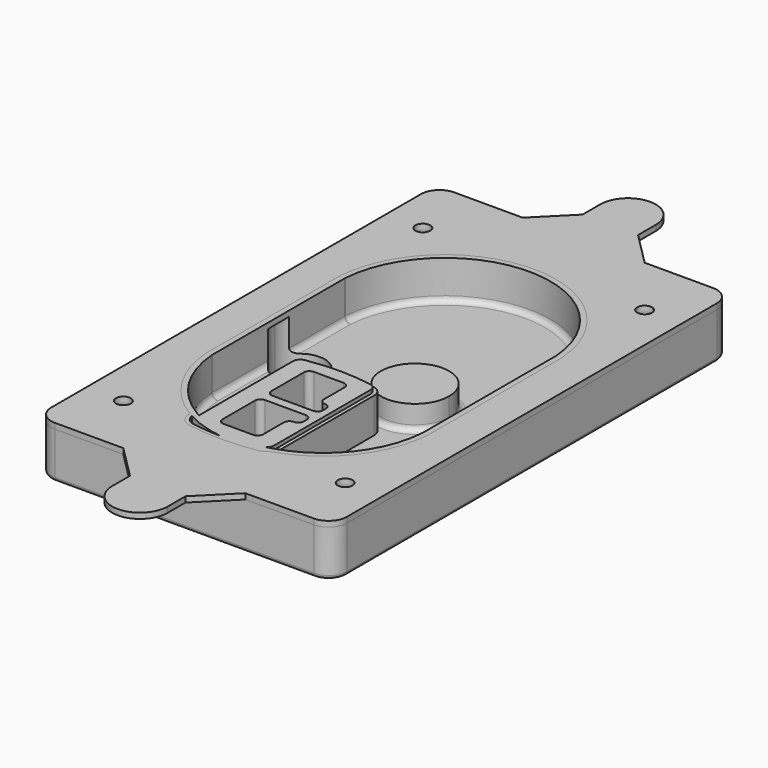
from build123d import *

# Parameters (mm, degrees)
F0_R      = 4
F1_DEPTH  = 25
F2_DEPTH  = 3
F3_DEPTH  = 18
F6_DEPTH  = 2
F8_DEPTH  = 20
F9_DEPTH  = 16
F10_DEPTH = 25
F7_R      = 6
F7_R_2    = 4
F11_DEPTH = 6
F13_DEPTH = 9
F14_R     = 3
F15_R     = 2
F16_R     = 4
F16_R_2   = 6
F17_DEPTH = 3


with BuildPart() as f1:
    # F0 (on Top) → F1 (new body)
    with BuildSketch(Plane.XY):
        with BuildLine():
            ThreePointArc((14.05, 38.3825811321), (16.9789321881, 31.3115133202), (24.05, 28.3825811321))
            Line((24.05, 28.3825811321), (164.05, 28.3825811321))
            ThreePointArc((164.05, 28.3825811321), (171.1210678119, 31.3115133202), (174.05, 38.3825811321))
            Line((174.05, 38.3825811321), (174.05, 288.3825811321))
            ThreePointArc((174.05, 288.3825811321), (171.1210678119, 295.4536489439), (164.05, 298.3825811321))
            Line((164.05, 298.3825811321), (24.05, 298.3825811321))
            ThreePointArc((24.05, 298.3825811321), (16.9789321881, 295.4536489439), (14.05, 288.3825811321))
            Line((14.05, 288.3825811321), (14.05, 38.3825811321))
        make_face()
        with Locations((34.05, 62.1325811321)):
            Circle(F0_R, mode=Mode.SUBTRACT)
        with Locations((154.05, 62.1325811321)):
            Circle(F0_R, mode=Mode.SUBTRACT)
        with Locations((34.05, 264.6325811321)):
            Circle(F0_R, mode=Mode.SUBTRACT)
        with BuildLine():
            ThreePointArc((30.05, 208.0453240566), (30.058730902, 208.5396812427), (30.0849127182, 209.033421831))
            ThreePointArc((30.0849127182, 209.033421831), (94.05, 268.6325811321), (158.0150872818, 209.033421831))
            ThreePointArc((158.0150872818, 209.033421831), (158.041269098, 208.5396812427), (158.05, 208.0453240566))
            Line((158.05, 208.0453240566), (158.05, 118.7198382075))
            ThreePointArc((158.05, 118.7198382075), (158.041269098, 118.2254810215), (158.0150872818, 117.7317404331))
            ThreePointArc((158.0150872818, 117.7317404331), (94.05, 58.1325811321), (30.0849127182, 117.7317404331))
            ThreePointArc((30.0849127182, 117.7317404331), (30.058730902, 118.2254810215), (30.05, 118.7198382075))
            Line((30.05, 118.7198382075), (30.05, 208.0453240566))
        make_face(mode=Mode.SUBTRACT)
        with Locations((154.05, 264.6325811321)):
            Circle(F0_R, mode=Mode.SUBTRACT)
        with BuildLine():
            ThreePointArc((158.0150872818, 209.033421831), (94.05, 268.6325811321), (30.0849127182, 209.033421831))
            ThreePointArc((30.0849127182, 209.033421831), (30.058730902, 208.5396812427), (30.05, 208.0453240566))
            Line((30.05, 208.0453240566), (30.05, 118.7198382075))
            ThreePointArc((30.05, 118.7198382075), (30.058730902, 118.2254810215), (30.0849127182, 117.7317404331))
            ThreePointArc((30.0849127182, 117.7317404331), (94.05, 58.1325811321), (158.0150872818, 117.7317404331))
            ThreePointArc((158.0150872818, 117.7317404331), (158.041269098, 118.2254810215), (158.05, 118.7198382075))
            Line((158.05, 118.7198382075), (158.05, 208.0453240566))
            ThreePointArc((158.05, 208.0453240566), (158.041269098, 208.5396812427), (158.0150872818, 209.033421831))
        make_face()
        with BuildLine():
            Line((34.05, 118.7198382075), (34.05, 208.0453240566))
            ThreePointArc((34.05, 208.0453240566), (34.0562363586, 208.3984363324), (34.0749376559, 208.7511081812))
            ThreePointArc((34.0749376559, 208.7511081812), (94.05, 264.6325811321), (154.0250623441, 208.7511081812))
            ThreePointArc((154.0250623441, 208.7511081812), (154.0437636414, 208.3984363324), (154.05, 208.0453240566))
            Line((154.05, 208.0453240566), (154.05, 118.7198382075))
            ThreePointArc((154.05, 118.7198382075), (154.0437636414, 118.3667259318), (154.0250623441, 118.0140540829))
            ThreePointArc((154.0250623441, 118.0140540829), (94.05, 62.1325811321), (34.0749376559, 118.0140540829))
            ThreePointArc((34.0749376559, 118.0140540829), (34.0562363586, 118.3667259318), (34.05, 118.7198382075))
        make_face(mode=Mode.SUBTRACT)
        with BuildLine():
            ThreePointArc((34.0749376559, 208.7511081812), (34.0562363586, 208.3984363324), (34.05, 208.0453240566))
            Line((34.05, 208.0453240566), (34.05, 118.7198382075))
            ThreePointArc((34.05, 118.7198382075), (34.0562363586, 118.3667259318), (34.0749376559, 118.0140540829))
            ThreePointArc((34.0749376559, 118.0140540829), (94.05, 62.1325811321), (154.0250623441, 118.0140540829))
            ThreePointArc((154.0250623441, 118.0140540829), (154.0437636414, 118.3667259318), (154.05, 118.7198382075))
            Line((154.05, 118.7198382075), (154.05, 208.0453240566))
            ThreePointArc((154.05, 208.0453240566), (154.0437636414, 208.3984363324), (154.0250623441, 208.7511081812))
            ThreePointArc((154.0250623441, 208.7511081812), (94.05, 264.6325811321), (34.0749376559, 208.7511081812))
        make_face()
        with BuildLine():
            ThreePointArc((151.0325436409, 208.5393729438), (151.045634549, 208.2925026496), (151.05, 208.0453240566))
            Line((151.05, 208.0453240566), (151.05, 118.7198382075))
            ThreePointArc((151.05, 118.7198382075), (151.045634549, 118.4726596145), (151.0325436409, 118.2257893203))
            ThreePointArc((151.0325436409, 118.2257893203), (94.05, 65.1325811321), (37.0674563591, 118.2257893203))
            ThreePointArc((37.0674563591, 118.2257893203), (37.054365451, 118.4726596145), (37.05, 118.7198382075))
            Line((37.05, 118.7198382075), (37.05, 208.0453240566))
            ThreePointArc((37.05, 208.0453240566), (37.054365451, 208.2925026496), (37.0674563591, 208.5393729438))
            ThreePointArc((37.0674563591, 208.5393729438), (94.05, 261.6325811321), (151.0325436409, 208.5393729438))
        make_face(mode=Mode.SUBTRACT)
        with BuildLine():
            Line((151.05, 118.7198382075), (151.05, 208.0453240566))
            ThreePointArc((151.05, 208.0453240566), (151.045634549, 208.2925026496), (151.0325436409, 208.5393729438))
            ThreePointArc((151.0325436409, 208.5393729438), (94.05, 261.6325811321), (37.0674563591, 208.5393729438))
            ThreePointArc((37.0674563591, 208.5393729438), (37.054365451, 208.2925026496), (37.05, 208.0453240566))
            Line((37.05, 208.0453240566), (37.05, 118.7198382075))
            ThreePointArc((37.05, 118.7198382075), (37.054365451, 118.4726596145), (37.0674563591, 118.2257893203))
            ThreePointArc((37.0674563591, 118.2257893203), (94.05, 65.1325811321), (151.0325436409, 118.2257893203))
            ThreePointArc((151.0325436409, 118.2257893203), (151.045634549, 118.4726596145), (151.05, 118.7198382075))
        make_face()
    extrude(amount=-F1_DEPTH)

    # F0 (on Top) → F2 (join)
    with BuildSketch(Plane.XY):
        with BuildLine():
            ThreePointArc((34.0749376559, 208.7511081812), (34.0562363586, 208.3984363324), (34.05, 208.0453240566))
            Line((34.05, 208.0453240566), (34.05, 118.7198382075))
            ThreePointArc((34.05, 118.7198382075), (34.0562363586, 118.3667259318), (34.0749376559, 118.0140540829))
            ThreePointArc((34.0749376559, 118.0140540829), (94.05, 62.1325811321), (154.0250623441, 118.0140540829))
            ThreePointArc((154.0250623441, 118.0140540829), (154.0437636414, 118.3667259318), (154.05, 118.7198382075))
            Line((154.05, 118.7198382075), (154.05, 208.0453240566))
            ThreePointArc((154.05, 208.0453240566), (154.0437636414, 208.3984363324), (154.0250623441, 208.7511081812))
            ThreePointArc((154.0250623441, 208.7511081812), (94.05, 264.6325811321), (34.0749376559, 208.7511081812))
        make_face()
        with BuildLine():
            ThreePointArc((151.0325436409, 208.5393729438), (151.045634549, 208.2925026496), (151.05, 208.0453240566))
            Line((151.05, 208.0453240566), (151.05, 118.7198382075))
            ThreePointArc((151.05, 118.7198382075), (151.045634549, 118.4726596145), (151.0325436409, 118.2257893203))
            ThreePointArc((151.0325436409, 118.2257893203), (94.05, 65.1325811321), (37.0674563591, 118.2257893203))
            ThreePointArc((37.0674563591, 118.2257893203), (37.054365451, 118.4726596145), (37.05, 118.7198382075))
            Line((37.05, 118.7198382075), (37.05, 208.0453240566))
            ThreePointArc((37.05, 208.0453240566), (37.054365451, 208.2925026496), (37.0674563591, 208.5393729438))
            ThreePointArc((37.0674563591, 208.5393729438), (94.05, 261.6325811321), (151.0325436409, 208.5393729438))
        make_face(mode=Mode.SUBTRACT)
    extrude(amount=F2_DEPTH)

    # F0 (on Top) → F3 (cut)
    with BuildSketch(Plane.XY):
        with BuildLine():
            Line((151.05, 118.7198382075), (151.05, 208.0453240566))
            ThreePointArc((151.05, 208.0453240566), (151.045634549, 208.2925026496), (151.0325436409, 208.5393729438))
            ThreePointArc((151.0325436409, 208.5393729438), (94.05, 261.6325811321), (37.0674563591, 208.5393729438))
            ThreePointArc((37.0674563591, 208.5393729438), (37.054365451, 208.2925026496), (37.05, 208.0453240566))
            Line((37.05, 208.0453240566), (37.05, 118.7198382075))
            ThreePointArc((37.05, 118.7198382075), (37.054365451, 118.4726596145), (37.0674563591, 118.2257893203))
            ThreePointArc((37.0674563591, 118.2257893203), (94.05, 65.1325811321), (151.0325436409, 118.2257893203))
            ThreePointArc((151.0325436409, 118.2257893203), (151.045634549, 118.4726596145), (151.05, 118.7198382075))
        make_face()
    extrude(amount=-F3_DEPTH, mode=Mode.SUBTRACT)

    # F4 (on face) → F5 (join, up to the next surface of F1)
    with BuildSketch(Plane.XY.offset(3)):
        with BuildLine():
            ThreePointArc((63.3, 70.0663530628), (65.1877495215, 64.9049197262), (69.9600985222, 62.1793597175))
            ThreePointArc((69.9600985222, 62.1793597175), (88.3, 60.6325811321), (106.6399014778, 62.1793597175))
            ThreePointArc((106.6399014778, 62.1793597175), (109.0997725506, 63.0263439319), (111.1577970177, 64.617847387))
            ThreePointArc((111.1577970177, 64.617847387), (98.7563887447, 62.3170645345), (86.1478631202, 62.6541260499))
            ThreePointArc((86.1478631202, 62.6541260499), (78.1937130529, 63.1086914432), (70.2950738916, 64.1511080538))
            ThreePointArc((70.2950738916, 64.1511080538), (66.9266219225, 65.9586086463), (65.3334610334, 69.4335712996))
            ThreePointArc((65.3334610334, 69.4335712996), (64.3111007877, 70.0023086838), (63.3, 70.5908304601))
            Line((63.3, 70.5908304601), (63.3, 70.0663530628))
        make_face()
        with BuildLine():
            ThreePointArc((107.5304157815, 66.7459245602), (109.1654742984, 67.168670617), (110.7873217221, 67.6395649966))
            ThreePointArc((110.7873217221, 67.6395649966), (111.1704314293, 68.826177739), (111.3, 70.0663530628))
            Line((111.3, 70.0663530628), (111.3, 135.1988092013))
            ThreePointArc((111.3, 135.1988092013), (109.8841878588, 139.0698842038), (106.3049261084, 141.1140542103))
            ThreePointArc((106.3049261084, 141.1140542103), (88.3, 142.6325811321), (70.2950738916, 141.1140542103))
            ThreePointArc((70.2950738916, 141.1140542103), (66.7158121412, 139.0698842038), (65.3, 135.1988092013))
            Line((65.3, 135.1988092013), (65.3, 72.8946079133))
            ThreePointArc((65.3, 72.8946079133), (66.2944325049, 72.3286907176), (67.3, 71.7828040152))
            Line((67.3, 71.7828040152), (67.3, 135.1988092013))
            ThreePointArc((67.3, 135.1988092013), (68.2438747608, 137.7795258696), (70.6300492611, 139.142305874))
            ThreePointArc((70.6300492611, 139.142305874), (88.3, 140.6325811321), (105.9699507389, 139.142305874))
            ThreePointArc((105.9699507389, 139.142305874), (108.3561252392, 137.7795258696), (109.3, 135.1988092013))
            Line((109.3, 135.1988092013), (109.3, 70.0663530628))
            ThreePointArc((109.3, 70.0663530628), (108.8299903064, 68.185085289), (107.5304157815, 66.7459245602))
        make_face()
        with BuildLine():
            ThreePointArc((67.3, 71.7828040152), (86.9533102792, 65.5751092381), (107.5304157815, 66.7459245602))
            ThreePointArc((107.5304157815, 66.7459245602), (108.8299903064, 68.185085289), (109.3, 70.0663530628))
            Line((109.3, 70.0663530628), (109.3, 135.1988092013))
            ThreePointArc((109.3, 135.1988092013), (108.3561252392, 137.7795258696), (105.9699507389, 139.142305874))
            ThreePointArc((105.9699507389, 139.142305874), (88.3, 140.6325811321), (70.6300492611, 139.142305874))
            ThreePointArc((70.6300492611, 139.142305874), (68.2438747608, 137.7795258696), (67.3, 135.1988092013))
            Line((67.3, 135.1988092013), (67.3, 71.7828040152))
        make_face()
        with BuildLine():
            Line((80.3, 100.1325811321), (102.3, 100.1325811321))
            ThreePointArc((102.3, 100.1325811321), (104.4213203436, 99.2539014756), (105.3, 97.1325811321))
            Line((105.3, 97.1325811321), (105.3, 95.1325811321))
            ThreePointArc((105.3, 95.1325811321), (104.4213203436, 93.0112607885), (102.3, 92.1325811321))
            ThreePointArc((102.3, 92.1325811321), (100.1786796564, 91.2539014756), (99.3, 89.1325811321))
            Line((99.3, 89.1325811321), (99.3, 75.1325811321))
            ThreePointArc((99.3, 75.1325811321), (98.4213203436, 73.0112607885), (96.3, 72.1325811321))
            Line((96.3, 72.1325811321), (80.3, 72.1325811321))
            ThreePointArc((80.3, 72.1325811321), (78.1786796564, 73.0112607885), (77.3, 75.1325811321))
            Line((77.3, 75.1325811321), (77.3, 97.1325811321))
            ThreePointArc((77.3, 97.1325811321), (78.1786796564, 99.2539014756), (80.3, 100.1325811321))
        make_face(mode=Mode.SUBTRACT)
        with BuildLine():
            ThreePointArc((80.3, 105.1325811321), (78.1786796564, 106.0112607885), (77.3, 108.1325811321))
            Line((77.3, 108.1325811321), (77.3, 130.1325811321))
            ThreePointArc((77.3, 130.1325811321), (78.1786796564, 132.2539014756), (80.3, 133.1325811321))
            Line((80.3, 133.1325811321), (96.3, 133.1325811321))
            ThreePointArc((96.3, 133.1325811321), (98.4213203436, 132.2539014756), (99.3, 130.1325811321))
            Line((99.3, 130.1325811321), (99.3, 116.1325811321))
            ThreePointArc((99.3, 116.1325811321), (100.1786796564, 114.0112607885), (102.3, 113.1325811321))
            ThreePointArc((102.3, 113.1325811321), (104.4213203436, 112.2539014756), (105.3, 110.1325811321))
            Line((105.3, 110.1325811321), (105.3, 108.1325811321))
            ThreePointArc((105.3, 108.1325811321), (104.4213203436, 106.0112607885), (102.3, 105.1325811321))
            Line((102.3, 105.1325811321), (80.3, 105.1325811321))
        make_face(mode=Mode.SUBTRACT)
    extrude(until=Until.NEXT, dir=(0, 0, -1))

    # F4 (on face) → F6 (cut)
    with BuildSketch(Plane.XY.offset(3)):
        with BuildLine():
            ThreePointArc((107.5304157815, 66.7459245602), (109.1654742984, 67.168670617), (110.7873217221, 67.6395649966))
            ThreePointArc((110.7873217221, 67.6395649966), (111.1704314293, 68.826177739), (111.3, 70.0663530628))
            Line((111.3, 70.0663530628), (111.3, 135.1988092013))
            ThreePointArc((111.3, 135.1988092013), (109.8841878588, 139.0698842038), (106.3049261084, 141.1140542103))
            ThreePointArc((106.3049261084, 141.1140542103), (88.3, 142.6325811321), (70.2950738916, 141.1140542103))
            ThreePointArc((70.2950738916, 141.1140542103), (66.7158121412, 139.0698842038), (65.3, 135.1988092013))
            Line((65.3, 135.1988092013), (65.3, 72.8946079133))
            ThreePointArc((65.3, 72.8946079133), (66.2944325049, 72.3286907176), (67.3, 71.7828040152))
            Line((67.3, 71.7828040152), (67.3, 135.1988092013))
            ThreePointArc((67.3, 135.1988092013), (68.2438747608, 137.7795258696), (70.6300492611, 139.142305874))
            ThreePointArc((70.6300492611, 139.142305874), (88.3, 140.6325811321), (105.9699507389, 139.142305874))
            ThreePointArc((105.9699507389, 139.142305874), (108.3561252392, 137.7795258696), (109.3, 135.1988092013))
            Line((109.3, 135.1988092013), (109.3, 70.0663530628))
            ThreePointArc((109.3, 70.0663530628), (108.8299903064, 68.185085289), (107.5304157815, 66.7459245602))
        make_face()
    extrude(amount=-F6_DEPTH, mode=Mode.SUBTRACT)

    # F7 (on face) → F8 (join)
    with BuildSketch(Plane(origin=(0, 0, -25), x_dir=(1, 0, 0), z_dir=(0, 0, -1))):
        with BuildLine():
            ThreePointArc((97.33842436, -163.3825811321), (110.8067035675, -149.9143019245), (124.274982775, -163.3825811321))
            Line((124.274982775, -163.3825811321), (129.274982775, -163.3825811321))
            ThreePointArc((129.274982775, -163.3825811321), (110.8067035675, -144.9143019245), (92.33842436, -163.3825811321))
            Line((92.33842436, -163.3825811321), (97.33842436, -163.3825811321))
        make_face()
        with BuildLine():
            Line((97.33842436, -163.3825811321), (124.274982775, -163.3825811321))
            ThreePointArc((124.274982775, -163.3825811321), (110.8067035675, -149.9143019245), (97.33842436, -163.3825811321))
        make_face()
        with BuildLine():
            ThreePointArc((97.33842436, -163.3825811321), (110.8067035675, -176.8508603396), (124.274982775, -163.3825811321))
            Line((124.274982775, -163.3825811321), (97.33842436, -163.3825811321))
        make_face()
        with BuildLine():
            Line((129.274982775, -163.3825811321), (124.274982775, -163.3825811321))
            ThreePointArc((124.274982775, -163.3825811321), (110.8067035675, -176.8508603396), (97.33842436, -163.3825811321))
            Line((97.33842436, -163.3825811321), (92.33842436, -163.3825811321))
            ThreePointArc((92.33842436, -163.3825811321), (110.8067035675, -181.8508603396), (129.274982775, -163.3825811321))
        make_face()
    extrude(amount=-F8_DEPTH)

    # F7 (on face) → F9 (cut)
    with BuildSketch(Plane(origin=(0, 0, -25), x_dir=(1, 0, 0), z_dir=(0, 0, -1))):
        with BuildLine():
            Line((97.33842436, -163.3825811321), (124.274982775, -163.3825811321))
            ThreePointArc((124.274982775, -163.3825811321), (110.8067035675, -149.9143019245), (97.33842436, -163.3825811321))
        make_face()
        with BuildLine():
            ThreePointArc((97.33842436, -163.3825811321), (110.8067035675, -176.8508603396), (124.274982775, -163.3825811321))
            Line((124.274982775, -163.3825811321), (97.33842436, -163.3825811321))
        make_face()
    extrude(amount=-F9_DEPTH, mode=Mode.SUBTRACT)

    # F7 (on face) → F10 (cut)
    with BuildSketch(Plane(origin=(0, 0, -25), x_dir=(1, 0, 0), z_dir=(0, 0, -1))):
        with BuildLine():
            Line((35.0181770675, -163.3825811321), (61.9547354825, -163.3825811321))
            ThreePointArc((61.9547354825, -163.3825811321), (48.486456275, -149.9143019245), (35.0181770675, -163.3825811321))
        make_face()
        with BuildLine():
            ThreePointArc((35.0181770675, -163.3825811321), (48.486456275, -176.8508603396), (61.9547354825, -163.3825811321))
            Line((61.9547354825, -163.3825811321), (35.0181770675, -163.3825811321))
        make_face()
    extrude(amount=-F10_DEPTH, mode=Mode.SUBTRACT)

    # F7 (on face) → F11 (cut)
    with BuildSketch(Plane(origin=(0, 0, -25), x_dir=(1, 0, 0), z_dir=(0, 0, -1))):
        with Locations((154.05, -264.6325811321)):
            Circle(F7_R)
        with Locations((154.05, -264.6325811321)):
            Circle(F7_R_2, mode=Mode.SUBTRACT)
        with Locations((34.05, -264.6325811321)):
            Circle(F7_R)
        with Locations((34.05, -264.6325811321)):
            Circle(F7_R_2, mode=Mode.SUBTRACT)
        with Locations((34.05, -62.1325811321)):
            Circle(F7_R)
        with Locations((34.05, -62.1325811321)):
            Circle(F7_R_2, mode=Mode.SUBTRACT)
        with Locations((154.05, -62.1325811321)):
            Circle(F7_R)
        with Locations((154.05, -62.1325811321)):
            Circle(F7_R_2, mode=Mode.SUBTRACT)
    extrude(amount=-F11_DEPTH, mode=Mode.SUBTRACT)

    # F12 (on face) → F13 (cut, through all)
    with BuildSketch(Plane(origin=(0, 0, -9), x_dir=(1, 0, 0), z_dir=(0, 0, -1))):
        with BuildLine():
            Line((99.3, -89.1325811321), (99.3, -100.1325811321))
            Line((99.3, -100.1325811321), (102.3, -100.1325811321))
            ThreePointArc((102.3, -100.1325811321), (104.4213203436, -99.2539014756), (105.3, -97.1325811321))
            Line((105.3, -97.1325811321), (105.3, -95.1325811321))
            ThreePointArc((105.3, -95.1325811321), (104.4213203436, -93.0112607885), (102.3, -92.1325811321))
            ThreePointArc((102.3, -92.1325811321), (100.1786796564, -91.2539014756), (99.3, -89.1325811321))
        make_face()
        with BuildLine():
            Line((102.3, -105.1325811321), (99.3, -105.1325811321))
            Line((99.3, -105.1325811321), (99.3, -116.1325811321))
            ThreePointArc((99.3, -116.1325811321), (100.1786796564, -114.0112607885), (102.3, -113.1325811321))
            ThreePointArc((102.3, -113.1325811321), (104.4213203436, -112.2539014756), (105.3, -110.1325811321))
            Line((105.3, -110.1325811321), (105.3, -108.1325811321))
            ThreePointArc((105.3, -108.1325811321), (104.4213203436, -106.0112607885), (102.3, -105.1325811321))
        make_face()
    extrude(amount=F13_DEPTH, mode=Mode.SUBTRACT)

    # F14
    f14_edges = [f1.edges().sort_by_distance(p)[0] for p in [
        (37.05, 137.494455, -18),
        (37.05, 189.270707, -18),
        (129.274983, 163.382581, -18),
        (45.560349, 92.057923, -18),
        (37.054365, 118.47266, -18),
        (37.054365, 208.292503, -18),
        (94.05, 261.632581, -18),
        (151.045635, 208.292503, -18),
        (151.05, 163.382581, -18),
        (151.045635, 118.47266, -18),
        (138.753424, 86.692578, -18),
    ]]
    fillet(f14_edges, radius=F14_R)

    # F15
    f15_edges = [f1.edges().sort_by_distance(p)[0] for p in [
        (94.05, 28.382581, -25),
        (14.05, 163.382581, -25),
        (16.978932, 295.453649, -25),
        (16.978932, 31.311513, -25),
        (94.05, 298.382581, -25),
        (171.121068, 295.453649, -25),
        (171.121068, 31.311513, -25),
        (174.05, 163.382581, -25),
    ]]
    fillet(f15_edges, radius=F15_R)


with BuildPart() as f17:
    # F16 (on face) → F17 (new body, through all)
    with BuildSketch(Plane.XY):
        with BuildLine():
            Line((164.05, 298.3825811321), (127.05, 298.3825811321))
            Line((127.05, 298.3825811321), (61.05, 298.3825811321))
            Line((61.05, 298.3825811321), (24.05, 298.3825811321))
            ThreePointArc((24.05, 298.3825811321), (16.9789321881, 295.4536489439), (14.05, 288.3825811321))
            Line((14.05, 288.3825811321), (14.05, 38.3825811321))
            ThreePointArc((14.05, 38.3825811321), (16.9789321881, 31.3115133202), (24.05, 28.3825811321))
            Line((24.05, 28.3825811321), (61.05, 28.3825811321))
            Line((61.05, 28.3825811321), (94.05, 28.3825811321))
            Line((94.05, 28.3825811321), (127.05, 28.3825811321))
            Line((127.05, 28.3825811321), (164.05, 28.3825811321))
            ThreePointArc((164.05, 28.3825811321), (171.1210678119, 31.3115133202), (174.05, 38.3825811321))
            Line((174.05, 38.3825811321), (174.05, 288.3825811321))
            ThreePointArc((174.05, 288.3825811321), (171.1210678119, 295.4536489439), (164.05, 298.3825811321))
        make_face()
        with Locations((34.05, 62.1325811321)):
            Circle(F16_R, mode=Mode.SUBTRACT)
        with Locations((154.05, 62.1325811321)):
            Circle(F16_R, mode=Mode.SUBTRACT)
        with BuildLine():
            ThreePointArc((34.05, 208.0453240566), (34.0562363586, 208.3984363324), (34.0749376559, 208.7511081812))
            ThreePointArc((34.0749376559, 208.7511081812), (94.05, 264.6325811321), (154.0250623441, 208.7511081812))
            ThreePointArc((154.0250623441, 208.7511081812), (154.0437636414, 208.3984363324), (154.05, 208.0453240566))
            Line((154.05, 208.0453240566), (154.05, 118.7198382075))
            ThreePointArc((154.05, 118.7198382075), (154.0437636414, 118.3667259318), (154.0250623441, 118.0140540829))
            ThreePointArc((154.0250623441, 118.0140540829), (140.9352911287, 84.6173752244), (111.1577970177, 64.617847387))
            ThreePointArc((111.1577970177, 64.617847387), (109.0997725506, 63.0263439319), (106.6399014778, 62.1793597175))
            ThreePointArc((106.6399014778, 62.1793597175), (88.3, 60.6325811321), (69.9600985222, 62.1793597175))
            ThreePointArc((69.9600985222, 62.1793597175), (65.1877495215, 64.9049197262), (63.3, 70.0663530628))
            Line((63.3, 70.0663530628), (63.3, 70.5908304601))
            ThreePointArc((63.3, 70.5908304601), (42.8640666879, 90.7137092079), (34.0749376559, 118.0140540829))
            ThreePointArc((34.0749376559, 118.0140540829), (34.0562363586, 118.3667259318), (34.05, 118.7198382075))
            Line((34.05, 118.7198382075), (34.05, 208.0453240566))
        make_face(mode=Mode.SUBTRACT)
        with Locations((34.05, 264.6325811321)):
            Circle(F16_R, mode=Mode.SUBTRACT)
        with Locations((154.05, 264.6325811321)):
            Circle(F16_R, mode=Mode.SUBTRACT)
        with BuildLine():
            Line((109.05, 10.3825811321), (127.05, 28.3825811321))
            Line((127.05, 28.3825811321), (94.05, 28.3825811321))
            Line((94.05, 28.3825811321), (61.05, 28.3825811321))
            Line((61.05, 28.3825811321), (79.05, 10.3825811321))
            Line((79.05, 10.3825811321), (79.05, -1.6174188679))
            ThreePointArc((79.05, -1.6174188679), (94.05, -16.6174188679), (109.05, -1.6174188679))
            Line((109.05, -1.6174188679), (109.05, 10.3825811321))
        make_face()
        with BuildLine():
            ThreePointArc((100.05, -1.6174188679), (89.8073593129, -5.8600595551), (94.05, 4.3825811321))
            ThreePointArc((94.05, 4.3825811321), (98.2926406871, 2.6252218192), (100.05, -1.6174188679))
        make_face(mode=Mode.SUBTRACT)
        with BuildLine():
            Line((127.05, 298.3825811321), (109.05, 316.3825811321))
            Line((109.05, 316.3825811321), (109.05, 328.3825811321))
            ThreePointArc((109.05, 328.3825811321), (94.05, 343.3825811321), (79.05, 328.3825811321))
            Line((79.05, 328.3825811321), (79.05, 316.3825811321))
            Line((79.05, 316.3825811321), (61.05, 298.3825811321))
            Line((61.05, 298.3825811321), (127.05, 298.3825811321))
        make_face()
        with Locations((94.05, 328.3825811321)):
            Circle(F16_R_2, mode=Mode.SUBTRACT)
        with Locations((94.05, 328.3825811321)):
            Circle(F16_R_2)
        with BuildLine():
            ThreePointArc((94.05, 4.3825811321), (89.8073593129, -5.8600595551), (100.05, -1.6174188679))
            ThreePointArc((100.05, -1.6174188679), (98.2926406871, 2.6252218192), (94.05, 4.3825811321))
        make_face()
    extrude(amount=F17_DEPTH)


solid = Compound([f1.part, f17.part])
